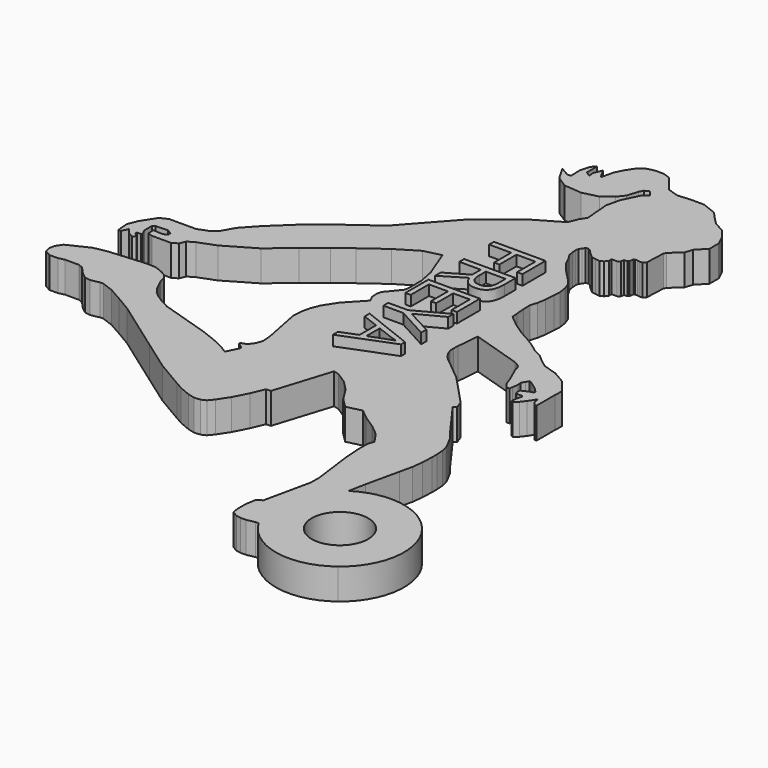
from build123d import *

# Parameters (mm, degrees)
F1_DEPTH     = 3
F2_R         = 2.75
F3_DEPTH     = 25
F4_TEXT_SIZE = 7.0322511925
F5_DEPTH     = 1


# Not quite as in the source:
# - Text() gives the source's letters only with a copy of the font that has no kerning and outlines rounded to 1/6400 em; it was checked with that copy


with BuildPart() as f1:
    # F0 (on Top) → F1 (new body)
    with BuildSketch(Plane.XY):
        with BuildLine():
            ThreePointArc((-9.1695703682, 3.5048335821), (-4.9962297782, 0.5269903975), (0, 1.6767772104))
            Line((0, 1.6767772104), (0, 11.6261636649))
            ThreePointArc((0, 11.6261636649), (-3.5256929745, 12.8914848465), (-7.1411709042, 11.9117563218))
            Line((-7.1411709042, 11.9117563218), (-6.8196714868, 13.5656509345))
            Line((-6.8196714868, 13.5656509345), (-6.0936631635, 16.8201699853))
            Line((-6.0936631635, 16.8201699853), (-5.8192266151, 18.0504024029))
            Line((-5.8192266151, 18.0504024029), (-5.6945736396, 19.101163631))
            Line((-5.6945736396, 19.101163631), (-5.6485189125, 20.188473165))
            Line((-5.6485189125, 20.188473165), (-5.6485189125, 20.7846630365))
            Line((-5.6485189125, 20.7846630365), (-5.7052988559, 21.5701181442))
            Line((-5.7052988559, 21.5701181442), (-5.827722236, 22.1098170287))
            Line((-5.827722236, 22.1098170287), (-6.1526680365, 22.7868873626))
            Line((-6.1526680365, 22.7868873626), (-6.5210303485, 23.4615510234))
            Line((-6.5210303485, 23.4615510234), (-7.3166675866, 24.5019979775))
            Line((-7.3166675866, 24.5019979775), (-9.602018632, 27.6596806943))
            Line((-9.602018632, 27.6596806943), (-9.3120308593, 27.8409216553))
            Line((-9.3120308593, 27.8409216553), (-9.5838941634, 28.6021400243))
            Line((-9.5838941634, 28.6021400243), (-12.4063845724, 31.6094649359))
            Line((-12.4063845724, 31.6094649359), (-14.2100593075, 33.0948457122))
            Line((-14.2100593075, 33.0948457122), (-14.691894874, 33.4709137678))
            Line((-14.691894874, 33.4709137678), (-15.1149705052, 33.8939912617))
            Line((-15.1149705052, 33.8939912617), (-15.3852691874, 34.3429413956))
            Line((-15.3852691874, 34.3429413956), (-15.5380470678, 34.7401425242))
            Line((-15.5380470678, 34.7401425242), (-15.5733032152, 35.2102257311))
            Line((-15.5733032152, 35.2102257311), (-15.5453154572, 35.7472945439))
            Line((-15.5453154572, 35.7472945439), (-15.3543108893, 37.8995587004))
            Line((-15.3543108893, 37.8995587004), (-10.5096586049, 36.3743901253))
            Line((-10.5096586049, 36.3743901253), (-9.9661322311, 36.0581576824))
            Line((-9.9661322311, 36.0581576824), (-9.7882505506, 35.7518047094))
            Line((-9.7882505506, 35.7518047094), (-9.72401537, 35.4454554617))
            Line((-9.72401537, 35.4454554617), (-9.0508256108, 33.9210703969))
            Line((-9.0508256108, 33.9210703969), (-8.7858531624, 33.1734679639))
            Line((-8.7858531624, 33.1734679639), (-8.3978567272, 32.7097661793))
            Line((-8.3978567272, 32.7097661793), (-8.1328833476, 32.7381566167))
            Line((-8.1328833476, 32.7381566167), (-8.0666402355, 33.0409817398))
            Line((-8.0666402355, 33.0409817398), (-8.0098602921, 33.5891954601))
            Line((-8.0098602921, 33.5891954601), (-8.0477138981, 33.9873172343))
            Line((-8.0477138981, 33.9873172343), (-7.840278894, 34.3429413956))
            Line((-7.840278894, 34.3429413956), (-7.6881074347, 34.6118956804))
            Line((-7.6881074347, 34.6118956804), (-7.460987661, 34.53892804))
            Line((-7.460987661, 34.53892804), (-6.656604819, 33.9589267969))
            Line((-6.656604819, 33.9589267969), (-6.2496820465, 33.533077687))
            Line((-6.2496820465, 33.533077687), (-6.2684080536, 33.3619141269))
            Line((-6.2684080536, 33.3619141269), (-6.6130902582, 33.2776069759))
            Line((-6.6130902582, 33.2776069759), (-6.9878213108, 33.0977626145))
            Line((-6.9878213108, 33.0977626145), (-7.2982353576, 32.949074577))
            Line((-7.2982353576, 32.949074577), (-7.3095741682, 32.681375742))
            Line((-7.3095741682, 32.681375742), (-7.2717210278, 32.4731841683))
            Line((-7.2717210278, 32.4731841683), (-7.0635280572, 32.3785506189))
            Line((-7.0635280572, 32.3785506189), (-6.6187516786, 32.3785506189))
            Line((-6.6187516786, 32.3785506189), (-6.5146549605, 32.2839170694))
            Line((-6.5146549605, 32.2839170694), (-6.5903617069, 32.0946499705))
            Line((-6.5903617069, 32.0946499705), (-6.694458425, 31.678263098))
            Line((-6.694458425, 31.678263098), (-6.7039215937, 31.2050972134))
            Line((-6.7039215937, 31.2050972134), (-6.5662250692, 31.1607165375))
            Line((-6.5662250692, 31.1607165375), (-6.171727553, 31.4755551517))
            Line((-6.171727553, 31.4755551517), (-5.80794253, 31.9410196226))
            Line((-5.80794253, 31.9410196226), (-5.3268231601, 32.6781327931))
            Line((-5.3268231601, 32.6781327931), (-5.2186938717, 32.1113415081))
            Line((-5.2186938717, 32.1113415081), (-4.9771065824, 31.8086290031))
            Line((-4.9771065824, 31.8086290031), (-4.7527219045, 31.8086290031))
            Line((-4.7527219045, 31.8086290031), (-4.7527219045, 33.5891954601))
            Line((-4.7527219045, 33.5891954601), (-4.7527219045, 34.0787072361))
            Line((-4.7527219045, 34.0787072361), (-4.7199880992, 34.8515221204))
            Line((-4.7199880992, 34.8515221204), (-4.9620391801, 35.1548157632))
            Line((-4.9620391801, 35.1548157632), (-5.7869866346, 36.1740318088))
            Line((-5.7869866346, 36.1740318088), (-6.9387214696, 36.8500800365))
            Line((-6.9387214696, 36.8500800365), (-8.3156879991, 37.2835695744))
            Line((-8.3156879991, 37.2835695744), (-8.8667003438, 37.6661978662))
            Line((-8.8667003438, 37.6661978662), (-9.7111649811, 38.3864454925))
            Line((-9.7111649811, 38.3864454925), (-10.566458106, 38.8365983963))
            Line((-10.566458106, 38.8365983963), (-11.2442327663, 39.354275912))
            Line((-11.2442327663, 39.354275912), (-12.0744742453, 39.8719534278))
            Line((-12.0744742453, 39.8719534278), (-13.0873210728, 40.4272192101))
            Line((-13.0873210728, 40.4272192101), (-14.3131399137, 41.2644454571))
            Line((-14.3131399137, 41.2644454571), (-15.3353656199, 42.1062792886))
            Line((-15.3353656199, 42.1062792886), (-15.3839240916, 42.7148673832))
            Line((-15.3839240916, 42.7148673832), (-15.4534041657, 43.5856679763))
            Line((-15.4534041657, 43.5856679763), (-15.4822040349, 44.3922206759))
            Line((-15.4822040349, 44.3922206759), (-15.2706662193, 45.0620912015))
            Line((-15.2706662193, 45.0620912015), (-15.1296406984, 45.8729863167))
            Line((-15.1296406984, 45.8729863167), (-15.0669082672, 46.8037200883))
            Line((-15.0669082672, 46.8037200883), (-15.036277473, 47.526884824))
            Line((-15.036277473, 47.526884824), (-15.1383540268, 48.224192995))
            Line((-15.1383540268, 48.224192995), (-15.3798384416, 48.9074542161))
            Line((-15.3798384416, 48.9074542161), (-15.7720074058, 49.4202896953))
            Line((-15.7720074058, 49.4202896953), (-16.3492690772, 49.9975532293))
            Line((-16.3492690772, 49.9975532293), (-16.9497173391, 50.6282894617))
            Line((-16.9497173391, 50.6282894617), (-17.6169704646, 51.4643676579))
            Line((-17.6169704646, 51.4643676579), (-17.9253316934, 52.1071858882))
            Line((-17.9253316934, 52.1071858882), (-18.3058636015, 52.7578287669))
            Line((-18.3058636015, 52.7578287669), (-18.3899750327, 53.2059517369))
            Line((-18.3899750327, 53.2059517369), (-18.4269491583, 53.6693520844))
            Line((-18.4269491583, 53.6693520844), (-18.377861008, 53.9393462241))
            Line((-18.377861008, 53.9393462241), (-18.2135691284, 54.1481237598))
            Line((-18.2135691284, 54.1481237598), (-18.0587768555, 54.4118322432))
            Line((-18.0587768555, 54.4118322432), (-17.8317371756, 54.4670596719))
            Line((-17.8317371756, 54.4670596719), (-17.6169704646, 54.3688796461))
            Line((-17.6169704646, 54.3688796461), (-17.3960663378, 54.1234314442))
            Line((-17.3960663378, 54.1234314442), (-17.0826535318, 53.8220107261))
            Line((-17.0826535318, 53.8220107261), (-16.7333576828, 53.5343550146))
            Line((-16.7333576828, 53.5343550146), (-16.3160953671, 53.4484498203))
            Line((-16.3160953671, 53.4484498203), (-15.9216813534, 53.4070691478))
            Line((-15.9216813534, 53.4070691478), (-15.5797498301, 53.5711720586))
            Line((-15.5797498301, 53.5711720586), (-15.3411160664, 53.8813563567))
            Line((-15.3411160664, 53.8813563567), (-15.3658632189, 54.1915148497))
            Line((-15.3658632189, 54.1915148497), (-14.8472916335, 54.1915148497))
            Line((-14.8472916335, 54.1915148497), (-14.6950744092, 54.2508549988))
            Line((-14.6950744092, 54.2508549988), (-14.587003374, 54.363962696))
            Line((-14.587003374, 54.363962696), (-14.532830897, 54.6673279053))
            Line((-14.532830897, 54.6673279053), (-14.2084318923, 54.6932112902))
            Line((-14.2084318923, 54.6932112902), (-14.0792311441, 54.7963231802))
            Line((-14.0792311441, 54.7963231802), (-14.0792311441, 55.0195003131))
            Line((-14.0792311441, 55.0195003131), (-14.0437707305, 55.218078196))
            Line((-14.0437707305, 55.218078196), (-13.9482785016, 55.2672279415))
            Line((-13.9482785016, 55.2672279415), (-13.6824406425, 55.2672279415))
            Line((-13.6824406425, 55.2672279415), (-13.4190926328, 55.2202014085))
            Line((-13.4190926328, 55.2202014085), (-13.1892475661, 55.2202014085))
            Line((-13.1892475661, 55.2202014085), (-13.0301588359, 55.3471661505))
            Line((-13.0301588359, 55.3471661505), (-12.9456110299, 55.4965995252))
            Line((-12.9456110299, 55.4965995252), (-12.8661180475, 57.3733553555))
            Line((-12.8661180475, 57.3733553555), (-12.7463769168, 57.618945837))
            Line((-12.7463769168, 57.618945837), (-11.7265548234, 58.54987674))
            Line((-11.7265548234, 58.54987674), (-11.4966481924, 59.2801682651))
            Line((-11.4966481924, 59.2801682651), (-10.6225472279, 60.1976774633))
            Line((-10.6225472279, 60.1976774633), (-10.6225472279, 61.3093575706))
            Line((-10.6225472279, 61.3093575706), (-11.0933779566, 62.2903996957))
            Line((-11.0933779566, 62.2903996957), (-11.7770303897, 63.1470264709))
            Line((-11.7770303897, 63.1470264709), (-12.840484269, 63.748717308))
            Line((-12.840484269, 63.748717308), (-13.3575769141, 64.2658099532))
            Line((-13.3575769141, 64.2658099532), (-14.0870366681, 65.062881357))
            Line((-14.0870366681, 65.062881357), (-15.4729560018, 65.6180021529))
            Line((-15.4729560018, 65.6180021529), (-16.8430483975, 65.6180021529))
            Line((-16.8430483975, 65.6180021529), (-18.0230045474, 65.5238549492))
            Line((-18.0230045474, 65.5238549492), (-19.0894609029, 65.8595912673))
            Line((-19.0894609029, 65.8595912673), (-19.8634099215, 66.8293610215))
            Line((-19.8634099215, 66.8293610215), (-20.3036729856, 67.3934593797))
            Line((-20.3036729856, 67.3934593797), (-21.0386198014, 67.6637589931))
            Line((-21.0386198014, 67.6637589931), (-21.8862599864, 67.667768265))
            Line((-21.8862599864, 67.667768265), (-22.645912967, 67.4819618101))
            Line((-22.645912967, 67.4819618101), (-23.260625166, 66.9913753579))
            Line((-23.260625166, 66.9913753579), (-23.7991297345, 66.1663434953))
            Line((-23.7991297345, 66.1663434953), (-24.159324596, 65.4275795558))
            Line((-24.159324596, 65.4275795558), (-24.4416768963, 64.2198621571))
            Line((-24.4416768963, 64.2198621571), (-24.9985232949, 65.1719719172))
            Line((-24.9985232949, 65.1719719172), (-25.3293207007, 64.4293384855))
            Line((-25.3293207007, 64.4293384855), (-25.2852365333, 63.8768272855))
            Line((-25.2852365333, 63.8768272855), (-25.7616522925, 64.1877874732))
            Line((-25.7616522925, 64.1877874732), (-25.7616522925, 64.6420270205))
            Line((-25.7616522925, 64.6420270205), (-25.7616522925, 65.4369443655))
            Line((-25.7616522925, 65.4369443655), (-26.1435862631, 65.0489479303))
            Line((-26.1435862631, 65.0489479303), (-26.3924250341, 64.1302310704))
            Line((-26.3924250341, 64.1302310704), (-26.3517796993, 62.9919410225))
            Line((-26.3517796993, 62.9919410225), (-26.723500242, 62.9919410225))
            Line((-26.723500242, 62.9919410225), (-27.6099086979, 63.5122473008))
            Line((-27.6099086979, 63.5122473008), (-26.8119592007, 62.147893493))
            Line((-26.8119592007, 62.147893493), (-25.7616522925, 61.4623501897))
            Line((-25.7616522925, 61.4623501897), (-24.0377116874, 61.3093575706))
            Line((-24.0377116874, 61.3093575706), (-22.5057099015, 61.6840758012))
            Line((-22.5057099015, 61.6840758012), (-21.5644907859, 62.4352392682))
            Line((-21.5644907859, 62.4352392682), (-21.0347126155, 63.0785406469))
            Line((-21.0347126155, 63.0785406469), (-20.7030263733, 64.1321320576))
            Line((-20.7030263733, 64.1321320576), (-20.5025887828, 64.5432319367))
            Line((-20.5025887828, 64.5432319367), (-20.0624913893, 64.7544475116))
            Line((-20.0624913893, 64.7544475116), (-19.6338576723, 64.2173630211))
            Line((-19.6338576723, 64.2173630211), (-20.1342973609, 63.8179746053))
            Line((-20.1342973609, 63.8179746053), (-20.4992152848, 63.0695236087))
            Line((-20.4992152848, 63.0695236087), (-20.9206094384, 62.2052391941))
            Line((-20.9206094384, 62.2052391941), (-21.2310755457, 60.8772694231))
            Line((-21.2310755457, 60.8772694231), (-21.0316644847, 58.3780310115))
            Line((-21.0316644847, 58.3780310115), (-21.4254988678, 57.7746453884))
            Line((-21.4254988678, 57.7746453884), (-21.7869616284, 56.8722143644))
            Line((-21.7869616284, 56.8722143644), (-24.5267539782, 55.2698324049))
            Line((-24.5267539782, 55.2698324049), (-27.9335648942, 52.5509417057))
            Line((-27.9335648942, 52.5509417057), (-32.1159766725, 47.8792339563))
            Line((-32.1159766725, 47.8792339563), (-34.8575658665, 45.8783269423))
            Line((-34.8575658665, 45.8783269423), (-37.5601574779, 43.7214560807))
            Line((-37.5601574779, 43.7214560807), (-39.6033786237, 41.7803935707))
            Line((-39.6033786237, 41.7803935707), (-40.847947384, 40.4272192101))
            Line((-40.847947384, 40.4272192101), (-41.5139049057, 39.2501776695))
            Line((-41.5139049057, 39.2501776695), (-42.1751067042, 38.7224890292))
            Line((-42.1751067042, 38.7224890292), (-43.1403666735, 38.3500234202))
            Line((-43.1403666735, 38.3500234202), (-45.759695904, 38.3500234202))
            Line((-45.759695904, 38.3500234202), (-46.4901637395, 37.9994506013))
            Line((-46.4901637395, 37.9994506013), (-47.3708631585, 36.6501489899))
            Line((-47.3708631585, 36.6501489899), (-47.7556379707, 35.6895168981))
            Line((-47.7556379707, 35.6895168981), (-47.663833946, 34.53892804))
            Line((-47.663833946, 34.53892804), (-47.4152456646, 34.53892804))
            Line((-47.4152456646, 34.53892804), (-47.1149608493, 35.1548157632))
            Line((-47.1149608493, 35.1548157632), (-46.7038491044, 34.6489981598))
            Line((-46.7038491044, 34.6489981598), (-46.1629114116, 34.3429413956))
            Line((-46.1629114116, 34.3429413956), (-45.9409342189, 34.6124848424))
            Line((-45.9409342189, 34.6124848424), (-46.3085023329, 34.9306483213))
            Line((-46.3085023329, 34.9306483213), (-46.2727248669, 35.0836807852))
            Line((-46.2727248669, 35.0836807852), (-45.8732469071, 35.0836807852))
            Line((-45.8732469071, 35.0836807852), (-45.8210890088, 35.1906572542))
            Line((-45.8210890088, 35.1906572542), (-46.0763902467, 35.7226133347))
            Line((-46.0763902467, 35.7226133347), (-46.0763902467, 36.6675445095))
            Line((-46.0763902467, 36.6675445095), (-45.8375625312, 36.8072241545))
            Line((-45.8375625312, 36.8072241545), (-44.6875492035, 36.8482880966))
            Line((-44.6875492035, 36.8482880966), (-44.2219777633, 36.5848727524))
            Line((-44.2219777633, 36.5848727524), (-44.2219777633, 36.2842356842))
            Line((-44.2219777633, 36.2842356842), (-44.6024858667, 36.1016187475))
            Line((-44.6024858667, 36.1016187475), (-45.5670006611, 36.160957964))
            Line((-45.5670006611, 36.160957964), (-45.518807512, 35.5569484939))
            Line((-45.518807512, 35.5569484939), (-45.0604185462, 35.3733438343))
            Line((-45.0604185462, 35.3733438343), (-43.2071737248, 35.3733438343))
            Line((-43.2071737248, 35.3733438343), (-42.6669987524, 35.6892680067))
            Line((-42.6669987524, 35.6892680067), (-42.4357036561, 36.2667213252))
            Line((-42.4357036561, 36.2667213252), (-41.7945459485, 36.6417057812))
            Line((-41.7945459485, 36.6417057812), (-40.1479266584, 37.2662842274))
            Line((-40.1479266584, 37.2662842274), (-37.3058840632, 38.9284677804))
            Line((-37.3058840632, 38.9284677804), (-35.0766070187, 40.795262903))
            Line((-35.0766070187, 40.795262903), (-33.1916846335, 42.2995723784))
            Line((-33.1916846335, 42.2995723784), (-31.6511280835, 43.4776470065))
            Line((-31.6511280835, 43.4776470065), (-29.4943451881, 45.0544543564))
            Line((-29.4943451881, 45.0544543564), (-27.4553128301, 46.2890696371))
            Line((-27.4553128301, 46.2890696371), (-25.8251105643, 46.6878071022))
            Line((-25.8251105643, 46.6878071022), (-24.7425119178, 43.904979463))
            Line((-24.7425119178, 43.904979463), (-24.4416768963, 42.38576442))
            Line((-24.4416768963, 42.38576442), (-24.4416768963, 40.9036498291))
            Line((-24.4416768963, 40.9036498291), (-24.5267539782, 40.4272192101))
            Line((-24.5267539782, 40.4272192101), (-25.114016307, 39.7141157136))
            Line((-25.114016307, 39.7141157136), (-25.6519569527, 39.0609027683))
            Line((-25.6519569527, 39.0609027683), (-25.7616522925, 38.5916982666))
            Line((-25.7616522925, 38.5916982666), (-25.7148750379, 38.0054343416))
            Line((-25.7148750379, 38.0054343416), (-25.4315435886, 37.4184437096))
            Line((-25.4315435886, 37.4184437096), (-27.0428671767, 35.7003794008))
            Line((-27.0428671767, 35.7003794008), (-27.8758071363, 34.4242490828))
            Line((-27.8758071363, 34.4242490828), (-28.2102823257, 33.5891954601))
            Line((-28.2102823257, 33.5891954601), (-28.3981841058, 32.7854752541))
            Line((-28.3981841058, 32.7854752541), (-28.4582819824, 31.8086290031))
            Line((-28.4582819824, 31.8086290031), (-28.2102823257, 30.5562322333))
            Line((-28.2102823257, 30.5562322333), (-27.9335648942, 29.158810874))
            Line((-27.9335648942, 29.158810874), (-27.7219232578, 28.090021887))
            Line((-27.7219232578, 28.090021887), (-27.6473767334, 27.1557229764))
            Line((-27.6473767334, 27.1557229764), (-27.8304216715, 26.5742862148))
            Line((-27.8304216715, 26.5742862148), (-28.0561708063, 26.2284205712))
            Line((-28.0561708063, 26.2284205712), (-28.2439804052, 26.0003663013))
            Line((-28.2439804052, 26.0003663013), (-28.5015612183, 25.8767457565))
            Line((-28.5015612183, 25.8767457565), (-28.7594637234, 25.8136643872))
            Line((-28.7594637234, 25.8136643872), (-28.8247779593, 25.6982252394))
            Line((-28.8247779593, 25.6982252394), (-28.2102823257, 25.1921694726))
            Line((-28.2102823257, 25.1921694726), (-28.8260819599, 23.9280651962))
            Line((-28.8260819599, 23.9280651962), (-29.4455699623, 24.3324097246))
            Line((-29.4455699623, 24.3324097246), (-30.6612681597, 24.925140664))
            Line((-30.6612681597, 24.925140664), (-32.1159766725, 25.4977665358))
            Line((-32.1159766725, 25.4977665358), (-34.7597886828, 26.330077868))
            Line((-34.7597886828, 26.330077868), (-35.9388663858, 26.7012690607))
            Line((-35.9388663858, 26.7012690607), (-36.9129561432, 27.0079270003))
            Line((-36.9129561432, 27.0079270003), (-37.7816783388, 27.463730037))
            Line((-37.7816783388, 27.463730037), (-38.4625234675, 27.9081228282))
            Line((-38.4625234675, 27.9081228282), (-38.9726497233, 28.3458549529))
            Line((-38.9726497233, 28.3458549529), (-39.3948127612, 28.9334252572))
            Line((-39.3948127612, 28.9334252572), (-39.6540915897, 29.4736692079))
            Line((-39.6540915897, 29.4736692079), (-39.8632626535, 29.9095065745))
            Line((-39.8632626535, 29.9095065745), (-40.0068350136, 30.4964892566))
            Line((-40.0068350136, 30.4964892566), (-40.3195576928, 30.924932998))
            Line((-40.3195576928, 30.924932998), (-40.787499398, 31.1896894127))
            Line((-40.787499398, 31.1896894127), (-41.5682010353, 31.5059237182))
            Line((-41.5682010353, 31.5059237182), (-42.4792293942, 31.5577623685))
            Line((-42.4792293942, 31.5577623685), (-43.6212894067, 31.4666388495))
            Line((-43.6212894067, 31.4666388495), (-44.8880758558, 31.3655635665))
            Line((-44.8880758558, 31.3655635665), (-46.1080059595, 31.2682268917))
            Line((-46.1080059595, 31.2682268917), (-47.3571337022, 31.0208745679))
            Line((-47.3571337022, 31.0208745679), (-48.363891928, 30.5377019325))
            Line((-48.363891928, 30.5377019325), (-49.3990045298, 30.040921205))
            Line((-49.3990045298, 30.040921205), (-49.7956462876, 29.4332344603))
            Line((-49.7956462876, 29.4332344603), (-49.8919015475, 28.8942061813))
            Line((-49.8919015475, 28.8942061813), (-49.7631286214, 28.3677296541))
            Line((-49.7631286214, 28.3677296541), (-49.1788424551, 28.0371467869))
            Line((-49.1788424551, 28.0371467869), (-48.3522933293, 28.0371467869))
            Line((-48.3522933293, 28.0371467869), (-47.7767065167, 28.1779317873))
            Line((-47.7767065167, 28.1779317873), (-47.0756404102, 28.1779317873))
            Line((-47.0756404102, 28.1779317873), (-46.3899669471, 28.1779317873))
            Line((-46.3899669471, 28.1779317873), (-45.9422618151, 27.9819983989))
            Line((-45.9422618151, 27.9819983989), (-45.4722943252, 27.4270435058))
            Line((-45.4722943252, 27.4270435058), (-44.7770837568, 26.8545165453))
            Line((-44.7770837568, 26.8545165453), (-44.1825695945, 26.7483530704))
            Line((-44.1825695945, 26.7483530704), (-43.3330796659, 26.9165690988))
            Line((-43.3330796659, 26.9165690988), (-43.0206470191, 26.9165690988))
            Line((-43.0206470191, 26.9165690988), (-41.8680710808, 26.4838172316))
            Line((-41.8680710808, 26.4838172316), (-40.6082296521, 25.7710124183))
            Line((-40.6082296521, 25.7710124183), (-39.1097776592, 24.8914472759))
            Line((-39.1097776592, 24.8914472759), (-34.0547524393, 21.2909597903))
            Line((-34.0547524393, 21.2909597903), (-31.0671757907, 19.1702414304))
            Line((-31.0671757907, 19.1702414304), (-28.4235943109, 17.6185052842))
            Line((-28.4235943109, 17.6185052842), (-27.6725403965, 17.1935670078))
            Line((-27.6725403965, 17.1935670078), (-26.602268219, 16.7400427163))
            Line((-26.602268219, 16.7400427163), (-25.9206593037, 16.5687669069))
            Line((-25.9206593037, 16.5687669069), (-25.318318978, 16.616826877))
            Line((-25.318318978, 16.616826877), (-24.8734155468, 16.8303490096))
            Line((-24.8734155468, 16.8303490096), (-24.4416768963, 17.3546025265))
            Line((-24.4416768963, 17.3546025265), (-23.7421505153, 18.4263326228))
            Line((-23.7421505153, 18.4263326228), (-23.0416171253, 19.783616066))
            Line((-23.0416171253, 19.783616066), (-22.5057099015, 21.072251969))
            Line((-22.5057099015, 21.072251969), (-22.0485524023, 21.072251969))
            Line((-22.0485524023, 21.072251969), (-20.3036729856, 26.6148091593))
            Line((-20.3036729856, 26.6148091593), (-19.7150823495, 26.4295120752))
            Line((-19.7150823495, 26.4295120752), (-18.6737893477, 25.7498522171))
            Line((-18.6737893477, 25.7498522171), (-17.7602488548, 24.8171724379))
            Line((-17.7602488548, 24.8171724379), (-16.8990726457, 23.4569922247))
            Line((-16.8990726457, 23.4569922247), (-16.0026401281, 22.5696805865))
            Line((-16.0026401281, 22.5696805865), (-14.5531305674, 22.9242217253))
            Line((-14.5531305674, 22.9242217253), (-13.6422710493, 22.1741013229))
            Line((-13.6422710493, 22.1741013229), (-12.4063845724, 21.3674288243))
            Line((-12.4063845724, 21.3674288243), (-11.4074554294, 20.5447804183))
            Line((-11.4074554294, 20.5447804183), (-10.6635289267, 19.4711461663))
            Line((-10.6635289267, 19.4711461663), (-10.8633143827, 18.8365336508))
            Line((-10.8633143827, 18.8365336508), (-10.8633143827, 17.6613219082))
            Line((-10.8633143827, 17.6613219082), (-10.7367706115, 16.0024571612))
            Line((-10.7367706115, 16.0024571612), (-10.2459741756, 12.2501878068))
            Line((-10.2459741756, 12.2501878068), (-10.2459741756, 11.2112881616))
            Line((-10.2459741756, 11.2112881616), (-11.2442327663, 6.6381318841))
            Line((-11.2442327663, 6.6381318841), (-11.7182918524, 6.3874585585))
            Line((-11.7182918524, 6.3874585585), (-11.8981112431, 5.3804721683))
            Line((-11.8981112431, 5.3804721683), (-11.8981112431, 4.2773367839))
            Line((-11.8981112431, 4.2773367839), (-11.7842940139, 3.7025604633))
            Line((-11.7842940139, 3.7025604633), (-11.2442327663, 3.3979553264))
            Line((-11.2442327663, 3.3979553264), (-10.817496106, 3.321752185))
            Line((-10.817496106, 3.321752185), (-10.2459741756, 3.321752185))
            Line((-10.2459741756, 3.321752185), (-9.4763245434, 3.4741582349))
            Line((-9.4763245434, 3.4741582349), (-9.1695703682, 3.5048335821))
        make_face()
        with BuildLine():
            Line((0, 11.6261636649), (0, 1.6767772104))
            ThreePointArc((0, 1.6767772104), (2.4697563247, 6.6514704376), (0, 11.6261636649))
        make_face()
    extrude(amount=F1_DEPTH)

    # F2 (on face) → F3 (cut)
    with BuildSketch(Plane.XY.offset(3)):
        with Locations((-3.7752462085, 6.6514704376)):
            Circle(F2_R)
    extrude(amount=-F3_DEPTH, mode=Mode.SUBTRACT)

    # F4 (on face) → F5 (join)
    with BuildSketch(Plane.XY.offset(3)):
        with Locations(Location((-22.9400377721, 50.0385314226), (0, 0, -90))):
            Text('FREYA', F4_TEXT_SIZE, font='Open Sans', text_align=(TextAlign.LEFT, TextAlign.BOTTOM))
    extrude(amount=F5_DEPTH)


solid = f1.part
